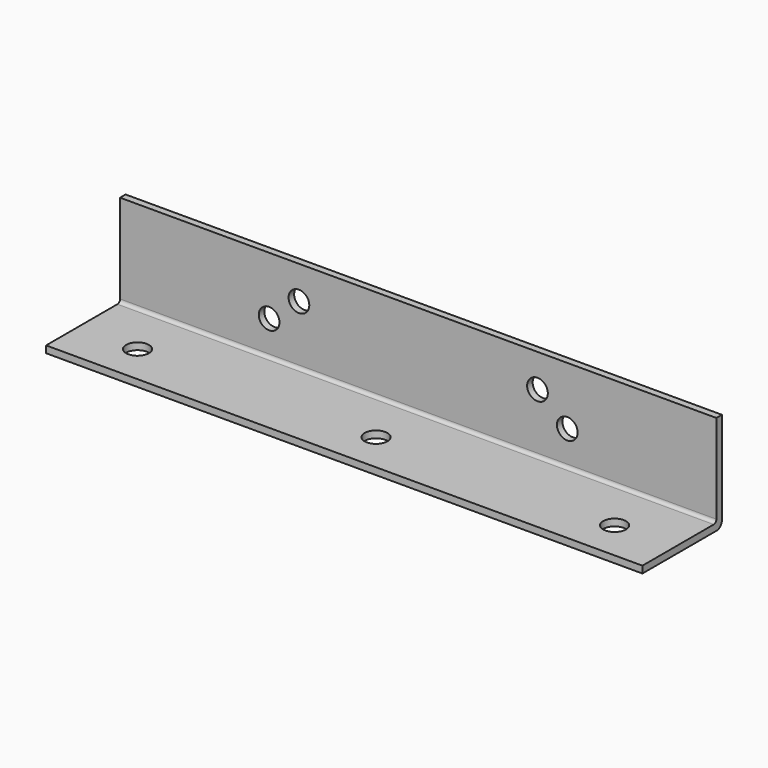
from build123d import *

# Parameters (mm, degrees)
F0_W     = 228.6
F0_H     = 38.1
F1_DEPTH = 2.65684
F2_W     = 228.6
F2_H     = 38.1
F3_DEPTH = 2.65684
F4_R     = 3.96875
F5_DEPTH = 2.65684
F6_R     = 4.365625
F7_DEPTH = 2.65684
F8_R     = 2.54
F9_R     = 1.27


# Not quite as in the source:
# - a pattern or mirror of a feature is missing from the dataset's text; its kind, count and spacing are read off the source's solid


with BuildPart() as f1:
    # F0 (on Front) → F1 (new body)
    with BuildSketch(Plane.XZ):
        Rectangle(F0_W, F0_H)
    extrude(amount=F1_DEPTH)

    # F2 (on face) → F3 (join)
    with BuildSketch(Plane(origin=(0, 0, -19.05), x_dir=(1, 0, 0), z_dir=(0, 0, -1))):
        with Locations((0, 19.05)):
            Rectangle(F2_W, F2_H)
    extrude(amount=-F3_DEPTH)

    # F4 (on face) → F5 (cut)
    with BuildSketch(Plane.XZ.offset(2.65684)):
        with Locations((-45.72, 6.35)):
            Circle(F4_R)
        with Locations((-57.15, -3.175)):
            Circle(F4_R)
    f5 = extrude(amount=-F5_DEPTH, mode=Mode.SUBTRACT)

    # F5_copies: F5 across plane
    add(f5.mirror(Plane(origin=(0, 0, 0), x_dir=(0, 0, 1), z_dir=(1, 0, 0))), mode=Mode.SUBTRACT)

    # F6 (on face) → F7 (cut)
    with BuildSketch(Plane(origin=(0, 0, -19.05), x_dir=(1, 0, 0), z_dir=(0, 0, -1))):
        with Locations((-91.44, 22.86)):
            Circle(F6_R)
        with Locations((0, 22.86)):
            Circle(F6_R)
        with Locations((91.44, 22.86)):
            Circle(F6_R)
    extrude(amount=-F7_DEPTH, mode=Mode.SUBTRACT)

    # F8
    f8_edges = [f1.edges().sort_by_distance(p)[0] for p in [
        (0, 0, -19.05),
    ]]
    fillet(f8_edges, radius=F8_R)

    # F9
    f9_edges = [f1.edges().sort_by_distance(p)[0] for p in [
        (0, -2.65684, -16.39316),
    ]]
    fillet(f9_edges, radius=F9_R)


solid = f1.part
